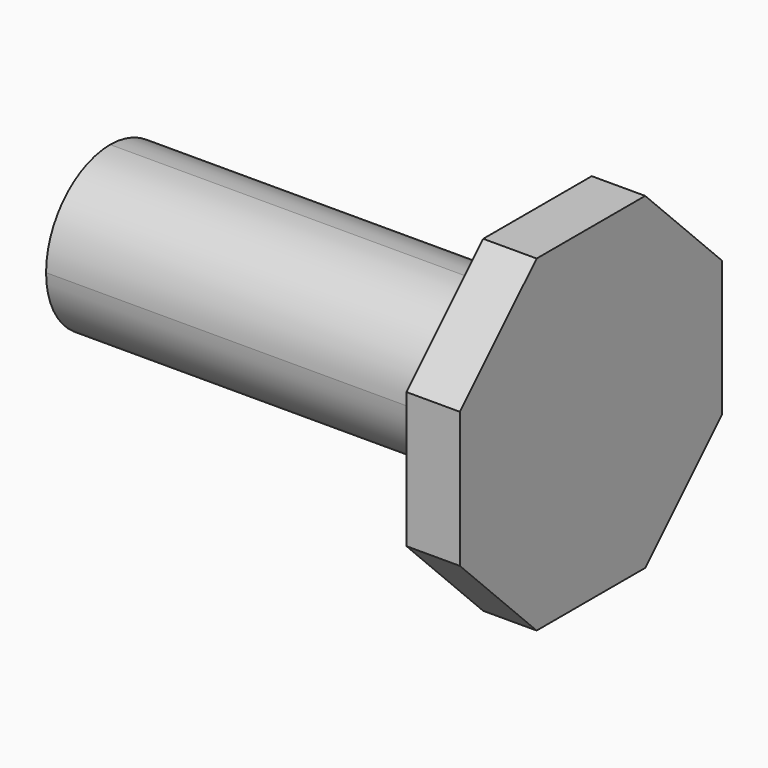
from build123d import *

# Parameters (mm, degrees)
F2_DEPTH = 5
F1_W     = 40
F1_H     = 15
F3_DEPTH = 7.5
F4_R     = 7.49999


# Not quite as in the source:
# - a fillet or chamfer is up to 0.001 mm smaller than in the source, because OpenCascade refuses the exact size


with BuildPart() as f2:
    # F0 (on Right) → F2 (new body)
    with BuildSketch(Plane.YZ):
        Polygon((15.3302561211, -6.35), (15.3302561211, 6.35), (6.35, 15.3302561211), (-6.35, 15.3302561211), (-15.3302561211, 6.35), (-15.3302561211, -6.35), (-6.35, -15.3302561211), (6.35, -15.3302561211), align=None)
    extrude(amount=F2_DEPTH)

    # F1 (on Top) → F3 (join, symmetric)
    with BuildSketch(Plane.XY):
        with Locations((-20, 0)):
            Rectangle(F1_W, F1_H)
    extrude(amount=F3_DEPTH, both=True)

    # F4 (radius 7.5 in the source; OpenCascade refuses exactly that, so slightly less here)
    f4_edges = [f2.edges().sort_by_distance(p)[0] for p in [
        (-20, 7.5, 7.5),
        (-20, 7.5, -7.5),
        (-20, -7.5, -7.5),
        (-20, -7.5, 7.5),
    ]]
    fillet(f4_edges, radius=F4_R)


solid = f2.part
